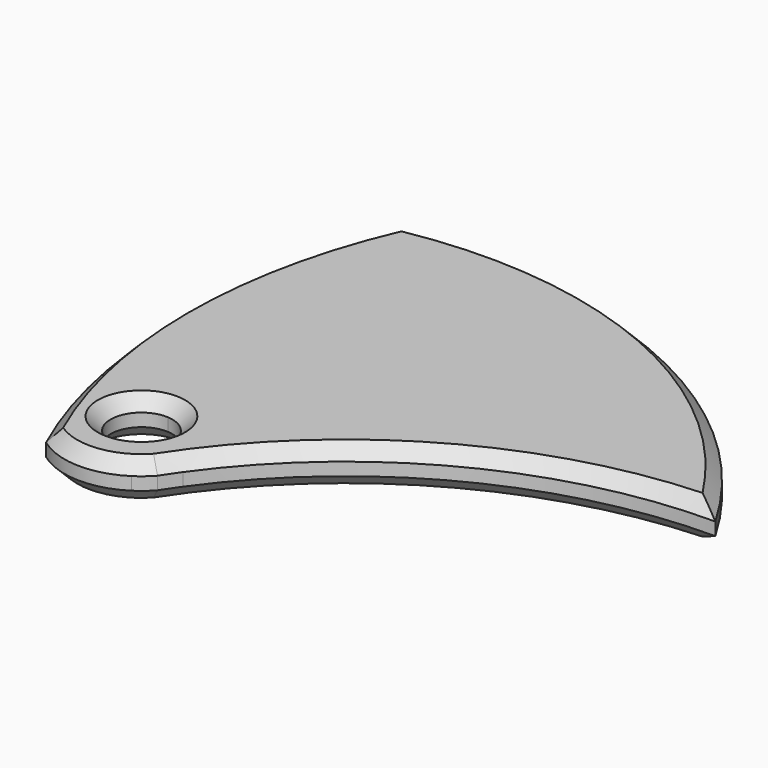
from build123d import *

# Parameters (mm, degrees)
F2_DEPTH     = 6.35
F3_T6_ANGLE  = 79.5586583167
F3_T8_ANGLE  = 79.5586583167
F3_T10_ANGLE = 63.5249338853
F3_T12_ANGLE = 63.5249338853
F3_T14_ANGLE = 109.1774772549
F3_T16_ANGLE = 109.1774772549
F3_T18_ANGLE = 50.5483837844
F3_T20_ANGLE = 50.5483837844


# Not quite as in the source:
# - a fillet or chamfer that OpenCascade refuses, or shapes differently, is made with other operations: its cross-section is extruded or revolved along the edge and cut away or added


with BuildPart() as f2:
    # F1 (on Top) → F2 (new body)
    with BuildSketch(Plane.XY):
        with BuildLine():
            ThreePointArc((-73.1568782646, -21.3192674026), (-75.6518657205, 9.1233334372), (-65.9911357684, 38.1))
            ThreePointArc((-65.9911357684, 38.1), (-73.5398929218, 37.7251690762), (-81.0143847835, 36.6043639223))
            ThreePointArc((-81.0143847835, 36.6043639223), (-88.9, 0), (-81.0143847835, -36.6043639223))
            ThreePointArc((-81.0143847835, -36.6043639223), (-73.8686107341, -39.0834183952), (-66.5806584514, -37.0601662189))
            ThreePointArc((-66.5806584514, -37.0601662189), (-68.3796387065, -33.6253626057), (-70.0015683829, -30.1034952113))
            ThreePointArc((-70.0015683829, -30.1034952113), (-78.2486807064, -28.1070619795), (-73.1568782646, -21.3192674026))
        make_face()
        with BuildLine():
            ThreePointArc((0, 0), (-27.8911357684, 27.8911357684), (-65.9911357684, 38.1))
            ThreePointArc((-65.9911357684, 38.1), (-75.6518657205, 9.1233334372), (-73.1568782646, -21.3192674026))
            ThreePointArc((-73.1568782646, -21.3192674026), (-69.7673746876, -22.9092911449), (-68.3877575616, -26.3897460844))
            ThreePointArc((-68.3877575616, -26.3897460844), (-68.8086460032, -28.4143644401), (-70.0015683829, -30.1034952113))
            ThreePointArc((-70.0015683829, -30.1034952113), (-68.3796387065, -33.6253626057), (-66.5806584514, -37.0601662189))
            ThreePointArc((-66.5806584514, -37.0601662189), (-65.2319724125, -36.0573126333), (-64.0275195551, -34.8851511001))
            ThreePointArc((-64.0275195551, -34.8851511001), (-63.0707476834, -33.4387934378), (-62.0813092162, -32.0145833333))
            ThreePointArc((-62.0813092162, -32.0145833333), (-34.925, -8.4749354005), (0, 0))
        make_face()
    extrude(amount=F2_DEPTH)

    # F3: chamfer of 2.1166666667 on 10 edges, made by hand

    # F3_s1 → F3_t2 (revolve, cut)
    with BuildSketch(Plane(origin=(-71.580679249, 4.3887278976, 0), x_dir=(0, 0, 1), z_dir=(-0.9981257248, 0.061196712, 0))):
        Polygon((4.2333333333, -25.7562696385), (6.35, -23.6396029718), (6.35, -25.7562696385), align=None)
    revolve(axis=Axis((-73.4677575616, -26.3897460844, 6.35), (0, 0, -1)), mode=Mode.SUBTRACT)

    # F3_s3 → F3_t4 (revolve, cut)
    with BuildSketch(Plane(origin=(-71.580679249, 4.3887278976, 0), x_dir=(0, 0, 1), z_dir=(-0.9981257248, 0.061196712, 0))):
        Polygon((0, -23.6396029718), (2.1166666667, -25.7562696385), (0, -25.7562696385), align=None)
    revolve(axis=Axis((-73.4677575616, -26.3897460844, 0), (0, 0, -1)), mode=Mode.SUBTRACT)

    # F3_s5 → F3_t6 (revolve, cut)
    with BuildSketch(Plane(origin=(2.3767752158, -4.8934699303, 0), x_dir=(0, 0, 1), z_dir=(0.4368960746, -0.8995119899, 0))):
        Polygon((4.2333333333, -0.1944417058), (6.35, 1.9222249609), (6.35, -0.1944417058), align=None)
    revolve(axis=Axis((-65.9911357684, -38.1, 6.35), (0, 0, 1)), revolution_arc=F3_T6_ANGLE, mode=Mode.SUBTRACT)

    # F3_s7 → F3_t8 (revolve, cut)
    with BuildSketch(Plane(origin=(2.3767752158, -4.8934699303, 0), x_dir=(0, 0, 1), z_dir=(0.4368960746, -0.8995119899, 0))):
        Polygon((0, 1.9222249609), (2.1166666667, -0.1944417058), (0, -0.1944417058), align=None)
    revolve(axis=Axis((-65.9911357684, -38.1, 0), (0, 0, 1)), revolution_arc=F3_T8_ANGLE, mode=Mode.SUBTRACT)

    # F3_s9 → F3_t10 (revolve, cut)
    with BuildSketch(Plane(origin=(-32.1255217702, -58.583184591, 0), x_dir=(0, 0, 1), z_dir=(-0.4808240877, -0.8768170828, 0))):
        Polygon((6.35, 41.6778711875), (4.2333333333, 39.5612045208), (6.35, 39.5612045208), align=None)
    revolve(axis=Axis((0, -76.2, 6.35), (0, 0, -1)), revolution_arc=F3_T10_ANGLE, mode=Mode.SUBTRACT)

    # F3_s11 → F3_t12 (revolve, cut)
    with BuildSketch(Plane(origin=(-32.1255217702, -58.583184591, 0), x_dir=(0, 0, 1), z_dir=(-0.4808240877, -0.8768170828, 0))):
        Polygon((0, 41.6778711875), (2.1166666667, 39.5612045208), (0, 39.5612045208), align=None)
    revolve(axis=Axis((0, -76.2, 0), (0, 0, -1)), revolution_arc=F3_T12_ANGLE, mode=Mode.SUBTRACT)

    # F3_s13 → F3_t14 (revolve, cut)
    with BuildSketch(Plane(origin=(-6.0616572407, 10.9442518524, 0), x_dir=(0, 0, 1), z_dir=(-0.484513618, 0.8747837184, 0))):
        Polygon((4.2333333333, -89.7545894961), (6.35, -87.6379228294), (6.35, -89.7545894961), align=None)
    revolve(axis=Axis((-73.4677575616, -26.3897460844, 6.35), (0, 0, 1)), revolution_arc=F3_T14_ANGLE, mode=Mode.SUBTRACT)

    # F3_s15 → F3_t16 (revolve, cut)
    with BuildSketch(Plane(origin=(-6.0616572407, 10.9442518524, 0), x_dir=(0, 0, 1), z_dir=(-0.484513618, 0.8747837184, 0))):
        Polygon((0, -87.6379228294), (2.1166666667, -89.7545894961), (0, -89.7545894961), align=None)
    revolve(axis=Axis((-73.4677575616, -26.3897460844, 0), (0, 0, 1)), revolution_arc=F3_T16_ANGLE, mode=Mode.SUBTRACT)

    # F3_s17 → F3_t18 (revolve, cut)
    with BuildSketch(Plane(origin=(0, 0, 0), x_dir=(0, 0, 1), z_dir=(0.4407105264, 0.8976492811, 0))):
        Polygon((4.2333333333, -88.9), (6.35, -86.7833333333), (6.35, -88.9), align=None)
    revolve(axis=Axis((0, 0, 6.35), (0, 0, 1)), revolution_arc=F3_T18_ANGLE, mode=Mode.SUBTRACT)

    # F3_s19 → F3_t20 (revolve, cut)
    with BuildSketch(Plane(origin=(0, 0, 0), x_dir=(0, 0, 1), z_dir=(0.4407105264, 0.8976492811, 0))):
        Polygon((2.1166666667, -88.9), (0, -86.7833333333), (0, -88.9), align=None)
    revolve(axis=Axis((0, 0, 0), (0, 0, 1)), revolution_arc=F3_T20_ANGLE, mode=Mode.SUBTRACT)


solid = f2.part
